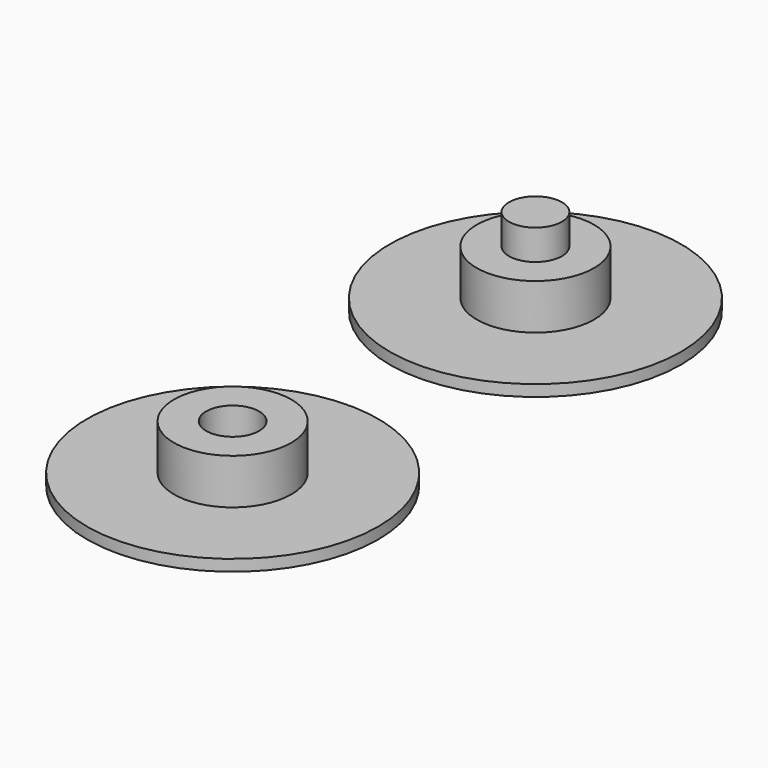
from build123d import *

# Parameters (mm, degrees)
F0_R     = 9.625
F0_R_2   = 3.875
F1_DEPTH = 0.75
F2_DEPTH = 3.75
F4_R     = 1.75
F5_DEPTH = 2
F6_DEPTH = 2


with BuildPart() as f1:
    # F0 (on Top) → F1 (new body)
    with BuildSketch(Plane.XY):
        Circle(F0_R)
        Circle(F0_R_2, mode=Mode.SUBTRACT)
    extrude(amount=F1_DEPTH)

    # F0 (on Top) → F2 (join)
    with BuildSketch(Plane.XY):
        Circle(F0_R_2)
    extrude(amount=F2_DEPTH)


with BuildPart() as f3_1:
    # F3: copy of F1
    add(f1.part.moved(Location((0, 25, 0))))

    # F4 (on face) → F5 (join)
    with BuildSketch(Plane.XY.offset(3.75)):
        with Locations((0, 25)):
            Circle(F4_R)
    extrude(amount=F5_DEPTH)


with BuildPart() as f1_1:
    add(f1.part)

    # F4 (on face) → F6 (cut)
    with BuildSketch(Plane.XY.offset(3.75)):
        Circle(F4_R)
    extrude(amount=-F6_DEPTH, mode=Mode.SUBTRACT)


solid = Compound([f3_1.part, f1_1.part])
